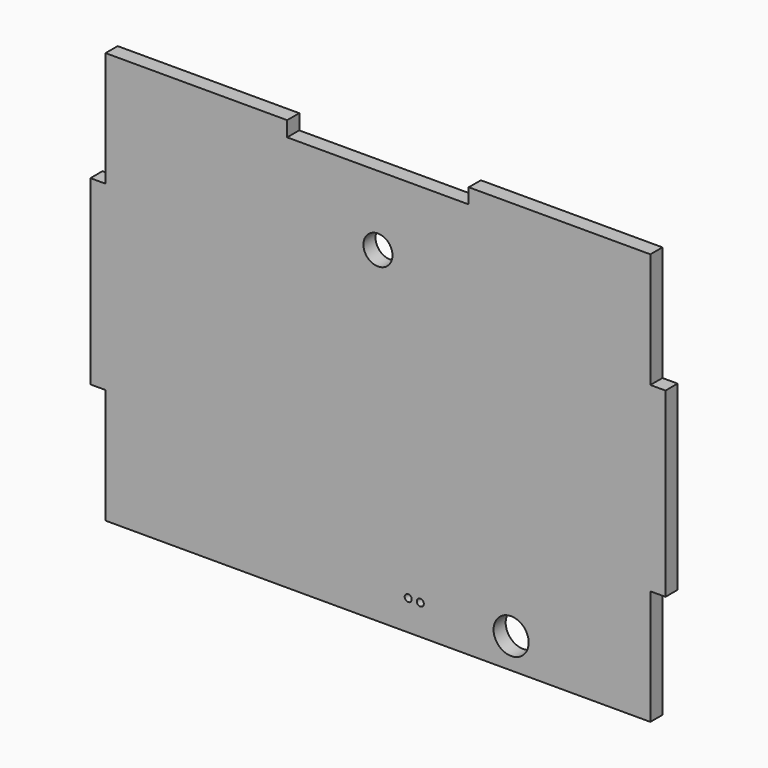
from build123d import *

# Parameters (mm, degrees)
F1_DEPTH = 3.175
F2_R     = 3.048
F2_R_2   = 3.683
F2_R_3   = 0.7366
F3_DEPTH = 3.176


# Not quite as in the source:
# - a feature names something its author has since deleted; it is built from what else it names


with BuildPart() as f1:
    # F0 (on Front) → F1 (new body)
    with BuildSketch(Plane.XZ):
        Polygon((-57.15, -43.18), (57.15, -43.18), (57.15, -19.05), (60.325, -19.05), (60.325, 19.05), (57.15, 19.05), (57.15, 43.18), (19.05, 43.18), (19.05, 40.005), (-19.05, 40.005), (-19.05, 43.18), (-57.15, 43.18), (-57.15, 19.05), (-60.325, 19.05), (-60.325, 0), (-60.325, -19.05), (-57.15, -19.05), align=None)
    extrude(amount=F1_DEPTH)

    # F2 (on face) → F3 (cut, through all)
    with BuildSketch(Plane.XZ.offset(3.175)):
        with Locations((0, 25.4)):
            Circle(F2_R)
        with Locations((27.94, -36.83)):
            Circle(F2_R_2)
        with Locations((6.35, -36.83)):
            Circle(F2_R_3)
        with Locations((8.89, -36.83)):
            Circle(F2_R_3)
    extrude(amount=-F3_DEPTH, mode=Mode.SUBTRACT)


solid = f1.part
